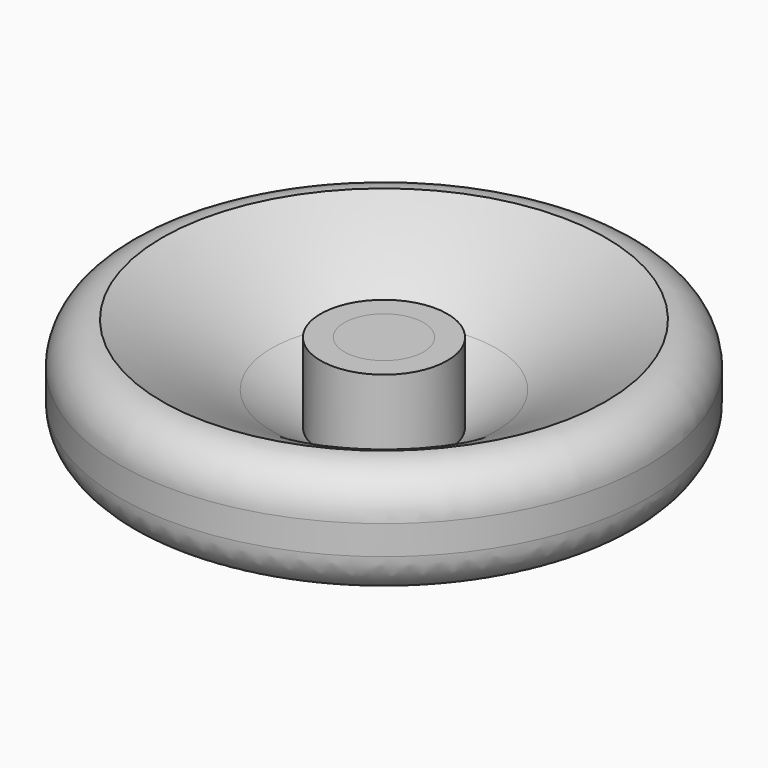
from build123d import *

# Parameters (mm, degrees)
F2_R     = 5.08
F4_R     = 213.36
F5_R     = 4.7625
F6_DEPTH = 9.525
F7_R     = 1.5875
F8_DEPTH = 8.89


# Not quite as in the source:
# - a fillet or chamfer that OpenCascade refuses, or shapes differently, is made with other operations: its cross-section is extruded or revolved along the edge and cut away or added


with BuildPart() as f1:
    # F0 (on Front) → F1 (revolve)
    with BuildSketch(Plane.XZ):
        Polygon((11.9791877568, 4.0159458295), (31.75, 8.134865202), (31.75, 20.834865202), (24.4433090497, 20.834865202), (7.62, 9.4384327507), (7.62, 18.9634327507), (0, 18.9634327507), (0, 0), align=None)
    revolve(axis=Axis((0, 0, 9.4817163754), (0, 0, -1)))

    # F2
    f2_edges = [f1.edges().sort_by_distance(p)[0] for p in [
        (-31.75, 0, 8.134865),
        (-31.75, 0, 20.834865),
        (31.75, 0, 14.484865),
    ]]
    fillet(f2_edges, radius=F2_R)

    # F3: fillet of radius 91.44 on 2 edges, made by hand

    # F3_s1 → F3_t2 (revolve, cut)
    with BuildSketch(Plane.XZ):
        with BuildLine():
            ThreePointArc((26.67, 20.834865202), (19.9318360713, 17.4009600318), (13.5004823618, 13.4219843706))
            Line((13.5004823618, 13.4219843706), (24.4433090497, 20.834865202))
            Line((24.4433090497, 20.834865202), (26.67, 20.834865202))
        make_face()
    revolve(axis=Axis((0, 0, 20.834865202), (0, 0, -1)), mode=Mode.SUBTRACT)

    # F4
    f4_edges = [f1.edges().sort_by_distance(p)[0] for p in [
        (-11.979188, 0, 4.015946),
        (-27.706088, 0, 7.292383),
    ]]
    fillet(f4_edges, radius=F4_R)


with BuildPart() as f6:
    # F5 (on face) → F6 (new body)
    with BuildSketch(Plane.XY.offset(18.9634327507)):
        Circle(F5_R)
    extrude(amount=-F6_DEPTH)


with BuildPart() as f8:
    # F7 (on Top) → F8 (new body)
    with BuildSketch(Plane.XY):
        Circle(F7_R)
    extrude(amount=F8_DEPTH)


solid = Compound([f1.part, f6.part, f8.part])
